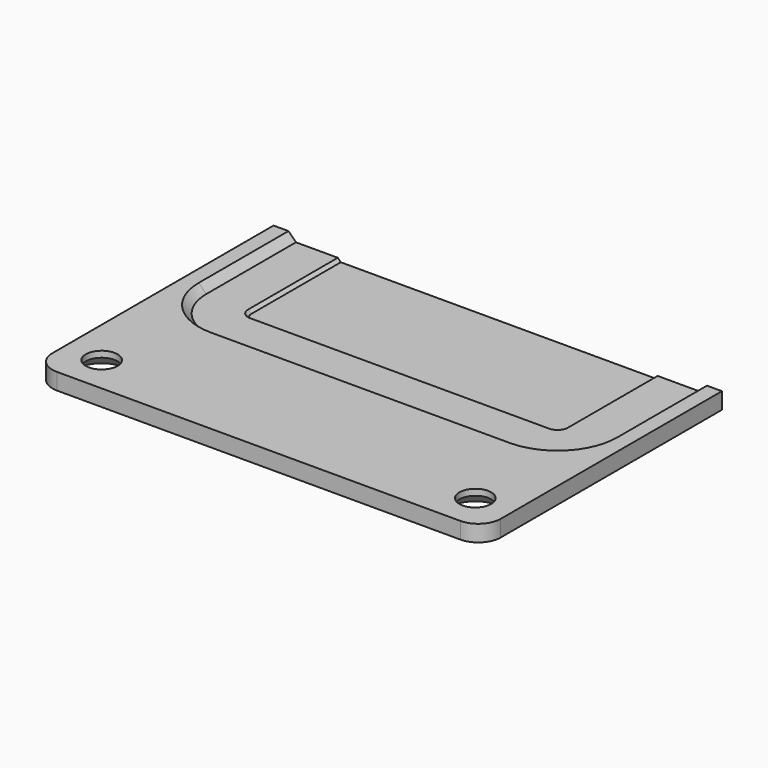
from build123d import *

# Parameters (mm, degrees)
F0_W           = 60
F0_H           = 40
F1_DEPTH       = 2.2
F2_D           = 4.25
F2_DEPTH       = 15
F2_CSINK_D     = 7
F2_CSINK_ANGLE = 90
F2_TIP         = 1.2768288154
F3_R           = 3
F4_W           = 50
F4_H           = 20
F5_DEPTH       = 1
F6_R           = 5
F7_T4_ANGLE    = 90
F7_T9_DEPTH    = 40
F7_T14_DEPTH   = 22.7150489639
F7_T19_ANGLE   = 90
F7_T24_DEPTH   = 22.7150489639
F9_DEPTH       = 0.4
F10_T4_ANGLE   = 90
F10_T9_DEPTH   = 40
F10_T14_DEPTH  = 15
F10_T19_ANGLE  = 90
F10_T24_DEPTH  = 15


# Not quite as in the source:
# - a fillet or chamfer that OpenCascade refuses, or shapes differently, is made with other operations: its cross-section is extruded or revolved along the edge and cut away or added


with BuildPart() as f1:
    # F0 (on Top) → F1 (new body)
    with BuildSketch(Plane.XY):
        Rectangle(F0_W, F0_H)
    extrude(amount=F1_DEPTH)

    # F2
    with Locations(Plane(origin=(0, 0, 0), x_dir=(1, 0, 0), z_dir=(0, 0, -1))):
        with Locations((-25, 15), (25, 15)):
            CounterSinkHole(F2_D / 2, F2_CSINK_D / 2, depth=F2_DEPTH, counter_sink_angle=F2_CSINK_ANGLE)
            with Locations((0, 0, -(F2_DEPTH + F2_TIP / 2))):  # 118° drill point
                Cone(0, F2_D / 2, F2_TIP, mode=Mode.SUBTRACT)

    # F3
    f3_edges = [f1.edges().sort_by_distance(p)[0] for p in [
        (-30, -20, 1.1),
        (30, -20, 1.1),
    ]]
    fillet(f3_edges, radius=F3_R)

    # F4 (on face) → F5 (cut)
    with BuildSketch(Plane.XY.offset(2.2)):
        with Locations((0, 10)):
            Rectangle(F4_W, F4_H)
    extrude(amount=-F5_DEPTH, mode=Mode.SUBTRACT)

    # F6
    f6_edges = [f1.edges().sort_by_distance(p)[0] for p in [
        (25, 0, 1.7),
        (-25, 0, 1.7),
    ]]
    fillet(f6_edges, radius=F6_R)

    # F7: chamfer of 3 on 1 edges, made by hand


with BuildPart() as f7_tool2:
    # F7_s3 → F7_t4 (revolve)
    with BuildSketch(Plane.YZ.offset(20)):
        Polygon((-3, 2.2), (0, -0.8), (0, 2.2), align=None)
    revolve(axis=Axis((20, 5, 2.2), (0, 0, 1)), revolution_arc=F7_T4_ANGLE)

    split(bisect_by=Plane.XY.offset(1.2), keep=Keep.TOP)


with BuildPart() as f1_1:
    add(f1.part)

    # F7_t1: cut F7_tool2
    add(f7_tool2.part, mode=Mode.SUBTRACT)


with BuildPart() as f7_tool7:
    # F7_s8 → F7_t9 (new body)
    with BuildSketch(Plane.YZ.offset(-20)):
        Polygon((-3, 2.2), (0, -0.8), (0, 2.2), align=None)
    extrude(amount=F7_T9_DEPTH)

    split(bisect_by=Plane.XY.offset(1.2), keep=Keep.TOP)


with BuildPart() as f1_2:
    add(f1_1.part)

    # F7_t6: cut F7_tool7
    add(f7_tool7.part, mode=Mode.SUBTRACT)


with BuildPart() as f7_tool12:
    # F7_s13 → F7_t14 (new body)
    with BuildSketch(Plane.XZ.offset(-5)):
        Polygon((28, 2.2), (25, -0.8), (25, 2.2), align=None)
    extrude(amount=-F7_T14_DEPTH)

    split(bisect_by=Plane.XY.offset(1.2), keep=Keep.TOP)


with BuildPart() as f1_3:
    add(f1_2.part)

    # F7_t11: cut F7_tool12
    add(f7_tool12.part, mode=Mode.SUBTRACT)


with BuildPart() as f7_tool17:
    # F7_s18 → F7_t19 (revolve)
    with BuildSketch(Plane.XZ.offset(-5)):
        Polygon((-28, 2.2), (-25, -0.8), (-25, 2.2), align=None)
    revolve(axis=Axis((-20, 5, 2.2), (0, 0, 1)), revolution_arc=F7_T19_ANGLE)

    split(bisect_by=Plane.XY.offset(1.2), keep=Keep.TOP)


with BuildPart() as f1_4:
    add(f1_3.part)

    # F7_t16: cut F7_tool17
    add(f7_tool17.part, mode=Mode.SUBTRACT)


with BuildPart() as f7_tool22:
    # F7_s23 → F7_t24 (new body)
    with BuildSketch(Plane.XZ.offset(-27.7150489639)):
        Polygon((-28, 2.2), (-25, -0.8), (-25, 2.2), align=None)
    extrude(amount=F7_T24_DEPTH)

    split(bisect_by=Plane.XY.offset(1.2), keep=Keep.TOP)


with BuildPart() as f1_5:
    add(f1_4.part)

    # F7_t21: cut F7_tool22
    add(f7_tool22.part, mode=Mode.SUBTRACT)

    # F8 (on face) → F9 (cut)
    with BuildSketch(Plane.XY.offset(1.2)):
        with BuildLine():
            ThreePointArc((20, 3), (21.4142135624, 3.5857864376), (22, 5))
            Line((22, 5), (22, 20))
            Line((22, 20), (-22, 20))
            Line((-22, 20), (-22, 5))
            ThreePointArc((-22, 5), (-21.4142135624, 3.5857864376), (-20, 3))
            Line((-20, 3), (20, 3))
        make_face()
    extrude(amount=-F9_DEPTH, mode=Mode.SUBTRACT)

    # F10: chamfer of 1 on 1 edges, made by hand


with BuildPart() as f10_tool2:
    # F10_s3 → F10_t4 (revolve)
    with BuildSketch(Plane.YZ.offset(20)):
        Polygon((4, 0.8), (3, 1.8), (3, 0.8), align=None)
    revolve(axis=Axis((20, 5, 0.8), (0, 0, 1)), revolution_arc=F10_T4_ANGLE)

    split(bisect_by=Plane.XY.offset(1.2), keep=Keep.BOTTOM)


with BuildPart() as f1_6:
    add(f1_5.part)

    # F10_t1: union F10_tool2
    add(f10_tool2.part)


with BuildPart() as f10_tool7:
    # F10_s8 → F10_t9 (new body)
    with BuildSketch(Plane.YZ.offset(-20)):
        Polygon((4, 0.8), (3, 1.8), (3, 0.8), align=None)
    extrude(amount=F10_T9_DEPTH)

    split(bisect_by=Plane.XY.offset(1.2), keep=Keep.BOTTOM)


with BuildPart() as f1_7:
    add(f1_6.part)

    # F10_t6: union F10_tool7
    add(f10_tool7.part)


with BuildPart() as f10_tool12:
    # F10_s13 → F10_t14 (new body)
    with BuildSketch(Plane.XZ.offset(-5)):
        Polygon((21, 0.8), (22, 1.8), (22, 0.8), align=None)
    extrude(amount=-F10_T14_DEPTH)

    split(bisect_by=Plane.XY.offset(1.2), keep=Keep.BOTTOM)


with BuildPart() as f1_8:
    add(f1_7.part)

    # F10_t11: union F10_tool12
    add(f10_tool12.part)


with BuildPart() as f10_tool17:
    # F10_s18 → F10_t19 (revolve)
    with BuildSketch(Plane.XZ.offset(-5)):
        Polygon((-21, 0.8), (-22, 1.8), (-22, 0.8), align=None)
    revolve(axis=Axis((-20, 5, 0.8), (0, 0, 1)), revolution_arc=F10_T19_ANGLE)

    split(bisect_by=Plane.XY.offset(1.2), keep=Keep.BOTTOM)


with BuildPart() as f1_9:
    add(f1_8.part)

    # F10_t16: union F10_tool17
    add(f10_tool17.part)


with BuildPart() as f10_tool22:
    # F10_s23 → F10_t24 (new body)
    with BuildSketch(Plane.XZ.offset(-20)):
        Polygon((-22, 1.8), (-21, 0.8), (-22, 0.8), align=None)
    extrude(amount=F10_T24_DEPTH)

    split(bisect_by=Plane.XY.offset(1.2), keep=Keep.BOTTOM)


with BuildPart() as f1_10:
    add(f1_9.part)

    # F10_t21: union F10_tool22
    add(f10_tool22.part)


solid = f1_10.part
